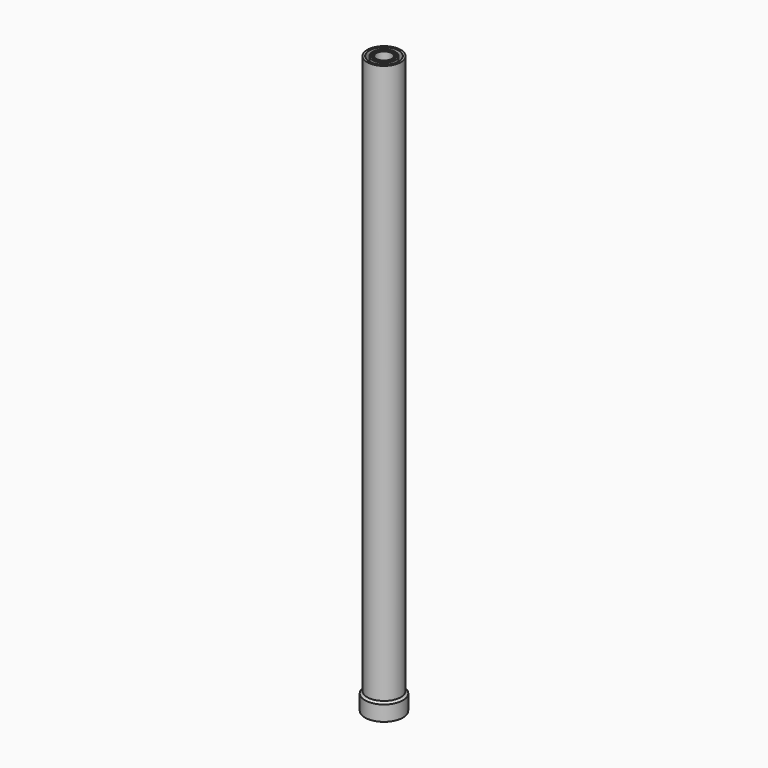
from build123d import *

# Parameters (mm, degrees)
F0_R      = 24.13
F0_R_2    = 20.447
F1_DEPTH  = 1524
F2_R      = 30.1625
F2_R_2    = 26.2509
F3_DEPTH  = 1524
F4_R      = 44.45
F4_R_2    = 38.9636
F5_DEPTH  = 1524
F8_R      = 0.396875
F11_R     = 0.396875
F14_R     = 0.396875
F15_DEPTH = 609.6
F16_DEPTH = 31.75


# Not quite as in the source:
# - a feature of the source that left no trace in its solid (it failed there, or was rolled back) is left out


with BuildPart() as f1:
    # F0 (on Top) → F1 (new body)
    with BuildSketch(Plane.XY):
        Circle(F0_R)
        Circle(F0_R_2, mode=Mode.SUBTRACT)
    extrude(amount=F1_DEPTH)


with BuildPart() as f3:
    # F2 (on Top) → F3 (new body)
    with BuildSketch(Plane.XY):
        Circle(F2_R)
        Circle(F2_R_2, mode=Mode.SUBTRACT)
    extrude(amount=F3_DEPTH)


with BuildPart() as f5:
    # F4 (on Top) → F5 (new body)
    with BuildSketch(Plane.XY):
        Circle(F4_R)
        Circle(F4_R_2, mode=Mode.SUBTRACT)
    extrude(amount=F5_DEPTH)


with BuildPart() as f7:
    # F6 (on Right) → F7 (revolve)
    with BuildSketch(Plane.YZ):
        Polygon((28.448, 50.8), (24.13, 50.8), (24.13, 33.02), (19.05, 26.67), (19.05, 24.13), (30.1625, 17.78), (30.1625, 0), (34.29, 0), (34.29, 20.6375), (28.448, 26.9875), align=None)
    revolve(axis=Axis((0, 0, 47.6393419911), (0, 0, 1)))

    # F8
    f8_edges = [f7.edges().sort_by_distance(p)[0] for p in [
        (0, -28.448, 50.8),
        (0, -28.448, 26.9875),
        (0, -34.29, 20.6375),
        (0, -19.05, 24.13),
        (0, -19.05, 26.67),
    ]]
    fillet(f8_edges, radius=F8_R)


with BuildPart() as f10:
    # F9 (on Right) → F10 (revolve)
    with BuildSketch(Plane.YZ):
        Polygon((44.45, 39.37), (44.45, 0), (50.165, 0), (50.165, 40.64), (34.544, 55.245), (34.544, 79.375), (30.1625, 79.375), (30.1625, 59.055), (25.4, 57.785), (25.4, 54.61), align=None)
    revolve(axis=Axis((0, 0, 51.9358633666), (0, 0, 1)))

    # F11
    f11_edges = [f10.edges().sort_by_distance(p)[0] for p in [
        (0, -50.165, 0),
        (0, -50.165, 40.64),
        (0, -34.544, 55.245),
        (0, -34.544, 79.375),
    ]]
    fillet(f11_edges, radius=F11_R)


with BuildPart() as f13:
    # F12 (on Right) → F13 (revolve)
    with BuildSketch(Plane.YZ):
        Polygon((34.925, 0), (34.925, 42.8625), (30.1625, 42.8625), (30.1625, 23.8125), (27.78125, 22.70125), (27.78125, 20.16125), (30.1625, 19.05), (30.1625, 0), align=None)
    revolve(axis=Axis((0, 0, 23.4007398409), (0, 0, 1)))

    # F14
    f14_edges = [f13.edges().sort_by_distance(p)[0] for p in [
        (0, -30.1625, 42.8625),
        (0, -34.925, 42.8625),
        (0, -34.925, 0),
        (0, -30.1625, 0),
    ]]
    fillet(f14_edges, radius=F14_R)


with BuildPart() as f15:
    # F2 (on Top) → F15 (new body)
    with BuildSketch(Plane.XY):
        Circle(F2_R)
        Circle(F2_R_2, mode=Mode.SUBTRACT)
    extrude(amount=F15_DEPTH)


with BuildPart() as f16:
    # F2 (on Top) → F16 (new body)
    with BuildSketch(Plane.XY):
        Circle(F2_R)
        Circle(F2_R_2, mode=Mode.SUBTRACT)
    extrude(amount=F16_DEPTH)


solid = Compound([f1.part, f3.part, f5.part, f7.part, f10.part, f13.part, f15.part, f16.part])
